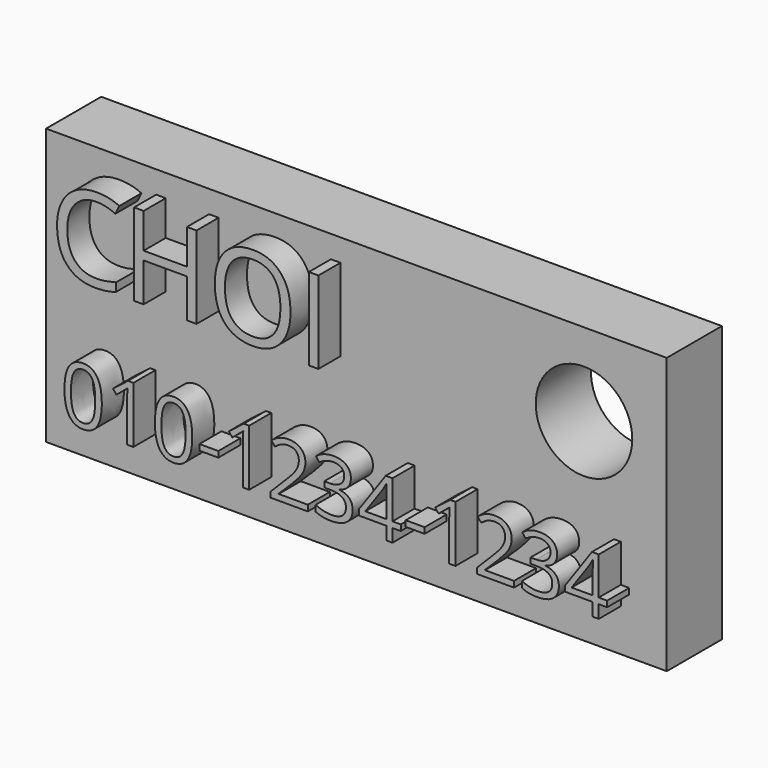
from build123d import *

# Parameters (mm, degrees)
F0_W         = 45
F0_H         = 20
F1_DEPTH     = 5
F2_TEXT_SIZE = 8.3561822692
F3_DEPTH     = 2
F4_TEXT_SIZE = 5.7329690509
F5_DEPTH     = 2
F6_R         = 3.5
F7_DEPTH     = 5


# Not quite as in the source:
# - Text() gives the source's letters only with a copy of the font that has no kerning and outlines rounded to 1/6400 em; it was checked with that copy


with BuildPart() as f1:
    # F0 (on Front) → F1 (new body)
    with BuildSketch(Plane.XZ):
        with Locations((22.5, 10)):
            Rectangle(F0_W, F0_H)
    extrude(amount=F1_DEPTH)

    # F2 (on face) → F3 (join)
    with BuildSketch(Plane.XZ.offset(5)):
        with Locations((1.8873701969, 12.4141547439)):
            Text('CHOI', F2_TEXT_SIZE, font='Open Sans', text_align=(TextAlign.LEFT, TextAlign.BOTTOM))
    extrude(amount=F3_DEPTH)

    # F4 (on face) → F5 (join)
    with BuildSketch(Plane.XZ.offset(5)):
        with Locations((2.6480338856, 3.0689439444)):
            Text('010-1234-1234', F4_TEXT_SIZE, font='Open Sans', text_align=(TextAlign.LEFT, TextAlign.BOTTOM))
    extrude(amount=F5_DEPTH)

    # F6 (on face) → F7 (cut)
    with BuildSketch(Plane.XZ.offset(5)):
        with Locations((39, 14)):
            Circle(F6_R)
    extrude(amount=-F7_DEPTH, mode=Mode.SUBTRACT)


solid = f1.part
